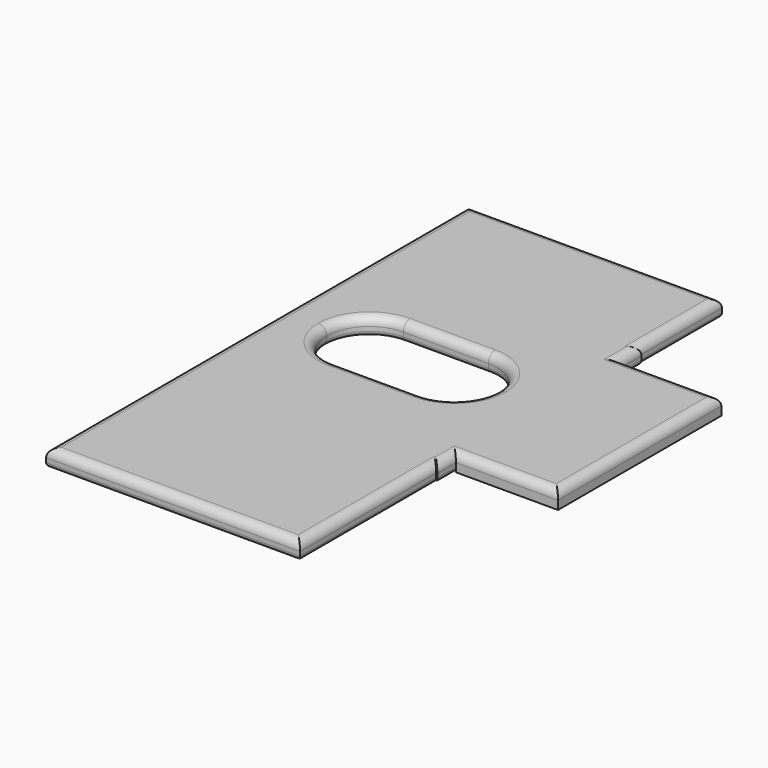
from build123d import *

# Parameters (mm, degrees)
F0_W     = 14.9271550402
F0_H     = 6
F0_H_2   = 10
F1_DEPTH = 1
F2_R     = 0.25
F3_DEPTH = 1
F0_W_2   = 6
F0_H_3   = 12
F4_DEPTH = 1
F5_R     = 0.5


# Not quite as in the source:
# - a feature names something its author has since deleted; it is built from what else it names


with BuildPart() as f1:
    # F0 (on Top) → F1 (new body)
    with BuildSketch(Plane.XY):
        with Locations((-0.0364224799, 10.5)):
            Rectangle(F0_W, F0_H)
        Polygon((7.4271550402, 7.5), (-7.5, 7.5), (-7.5, -7.5), (7.4271550402, -7.5), (7.5, -7.5), (7.5, -6.1350027099), (7.5, 5.8649972901), (7.5, 7.5), align=None)
        with BuildLine():
            ThreePointArc((-5, 0), (-4.267766953, 1.767766953), (-2.5, 2.5))
            Line((-2.5, 2.5), (2.5, 2.5))
            ThreePointArc((2.5, 2.5), (4.267766953, 1.767766953), (5, 0))
            ThreePointArc((5, 0), (4.267766953, -1.767766953), (2.5, -2.5))
            Line((2.5, -2.5), (-2.5, -2.5))
            ThreePointArc((-2.5, -2.5), (-4.267766953, -1.767766953), (-5, 0))
        make_face(mode=Mode.SUBTRACT)
        with Locations((-0.0364224799, -12.5)):
            Rectangle(F0_W, F0_H_2)
    extrude(amount=F1_DEPTH)

    # F2
    f2_edges = [f1.edges().sort_by_distance(p)[0] for p in [
        (-0.036422, 13.5, 0),
        (-7.5, -2, 0),
        (-0.036422, -17.5, 0),
        (7.427155, -12.5, 0),
        (7.463578, -7.5, 0),
        (7.5, 0, 0),
        (7.463578, 7.5, 0),
        (7.427155, 10.5, 0),
        (-5, 0, 0),
        (0, 2.5, 0),
        (5, 0, 0),
        (0, -2.5, 0),
    ]]
    fillet(f2_edges, radius=F2_R)

    # F0 (on Top) → F3 (cut)
    with BuildSketch(Plane.XY):
        with BuildLine():
            Line((2.5, 2.5), (-2.5, 2.5))
            ThreePointArc((-2.5, 2.5), (-4.267766953, 1.767766953), (-5, 0))
            ThreePointArc((-5, 0), (-4.267766953, -1.767766953), (-2.5, -2.5))
            Line((-2.5, -2.5), (2.5, -2.5))
            ThreePointArc((2.5, -2.5), (4.267766953, -1.767766953), (5, 0))
            ThreePointArc((5, 0), (4.267766953, 1.767766953), (2.5, 2.5))
        make_face()
    extrude(amount=F3_DEPTH, mode=Mode.SUBTRACT)

    # F0 (on Top) → F4 (join)
    with BuildSketch(Plane.XY):
        with Locations((10.5, -0.1350027099)):
            Rectangle(F0_W_2, F0_H_3)
    extrude(amount=F4_DEPTH)

    # F5
    f5_edges = [f1.edges().sort_by_distance(p)[0] for p in [
        (-0.036422, 13.5, 1),
        (-7.5, -2, 1),
        (-0.036422, -17.5, 1),
        (7.427155, -12.5, 1),
        (7.463578, -7.5, 1),
        (7.5, -6.817501, 1),
        (10.5, -6.135003, 1),
        (13.5, -0.135003, 1),
        (10.5, 5.864997, 1),
        (7.5, 6.682499, 1),
        (7.463578, 7.5, 1),
        (7.427155, 10.5, 1),
        (-5, 0, 1),
        (0, 2.5, 1),
        (5, 0, 1),
        (0, -2.5, 1),
    ]]
    fillet(f5_edges, radius=F5_R)


solid = f1.part
